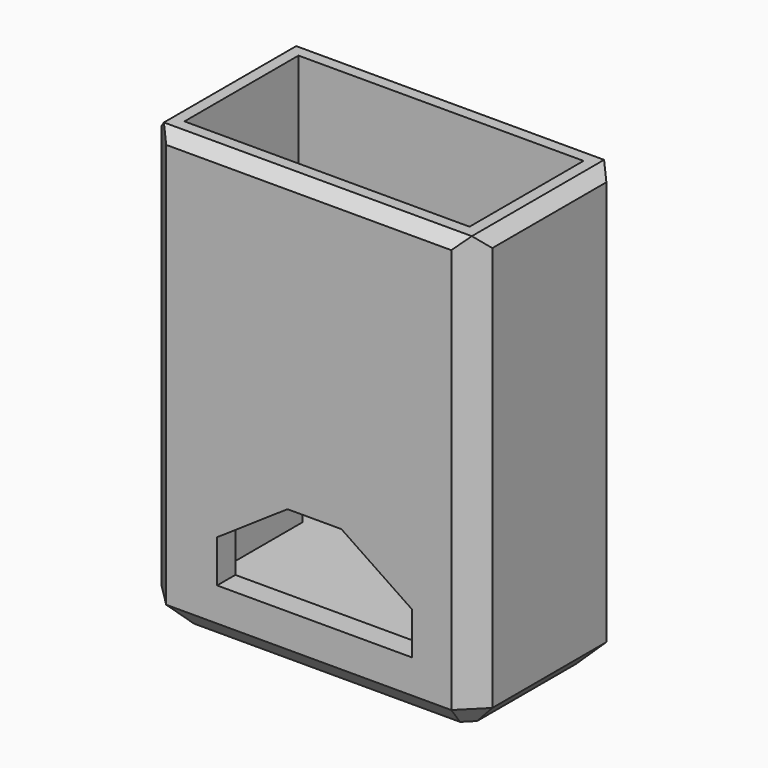
from build123d import *

# Parameters (mm, degrees)
F0_W      = 29
F0_H      = 16.5
F1_DEPTH  = 38.5
F2_T      = -2
F3_DEPTH  = 2.25
F4_SIZE   = 2
F5_SIZE   = 2
F6_SIZE   = 0.99999
F8_DEPTH  = 16.501
F9_W      = 7.54
F9_H      = 7.25
F9_R      = 1.1
F10_DEPTH = 4.35


# Not quite as in the source:
# - a fillet or chamfer is up to 0.001 mm smaller than in the source, because OpenCascade refuses the exact size


with BuildPart() as f1:
    # F0 (on Top) → F1 (new body)
    with BuildSketch(Plane.XY):
        with Locations((14.5, 8.25)):
            Rectangle(F0_W, F0_H)
    extrude(amount=-F1_DEPTH)

    # F2
    f2_openings = [f1.faces().sort_by_distance(p)[0] for p in [
        (14.5, 8.25, 0),
    ]]
    offset(amount=F2_T, openings=f2_openings)

    # F3 (add): a face of the model
    f3_faces = [f1.faces().sort_by_distance(p)[0] for p in [
        (14.5, 8.25, -36.5),
    ]]
    extrude(f3_faces, amount=F3_DEPTH)

    # F4
    f4_edges = [f1.edges().sort_by_distance(p)[0] for p in [
        (29, 0, -19.25),
        (0, 0, -19.25),
        (0, 16.5, -19.25),
        (29, 16.5, -19.25),
    ]]
    chamfer(f4_edges, length=F4_SIZE)

    # F5
    f5_edges = [f1.edges().sort_by_distance(p)[0] for p in [
        (0, 8.25, -38.5),
        (1, 15.5, -38.5),
        (1, 1, -38.5),
        (14.5, 16.5, -38.5),
        (14.5, 0, -38.5),
        (28, 15.5, -38.5),
        (28, 1, -38.5),
        (29, 8.25, -38.5),
    ]]
    chamfer(f5_edges, length=F5_SIZE)

    # F6 (size 1 in the source; OpenCascade refuses exactly that, so slightly less here)
    f6_edges = [f1.edges().sort_by_distance(p)[0] for p in [
        (0, 8.25, 0),
        (14.5, 16.5, 0),
        (29, 8.25, 0),
        (14.5, 0, 0),
    ]]
    chamfer(f6_edges, length=F6_SIZE)

    # F7 (on face) → F8 (cut, through all)
    with BuildSketch(Plane.XZ):
        Polygon((23.536, -33.56), (23.536, -29.836), (17.365, -25.666), (12.635, -25.666), (6.464, -29.836), (6.464, -33.56), align=None)
    extrude(amount=-F8_DEPTH, mode=Mode.SUBTRACT)

    # F9 (on face) → F10 (join)
    with BuildSketch(Plane(origin=(0, 0, 0), x_dir=(0, -1, 0), z_dir=(-1, 0, 0))):
        with Locations((-8.25, -30.625)):
            Rectangle(F9_W, F9_H)
        with Locations((-8.25, -29.5)):
            Circle(F9_R, mode=Mode.SUBTRACT)
        with Locations((-8.25, -29.5)):
            Circle(F9_R)
    extrude(amount=-F10_DEPTH)


solid = f1.part
